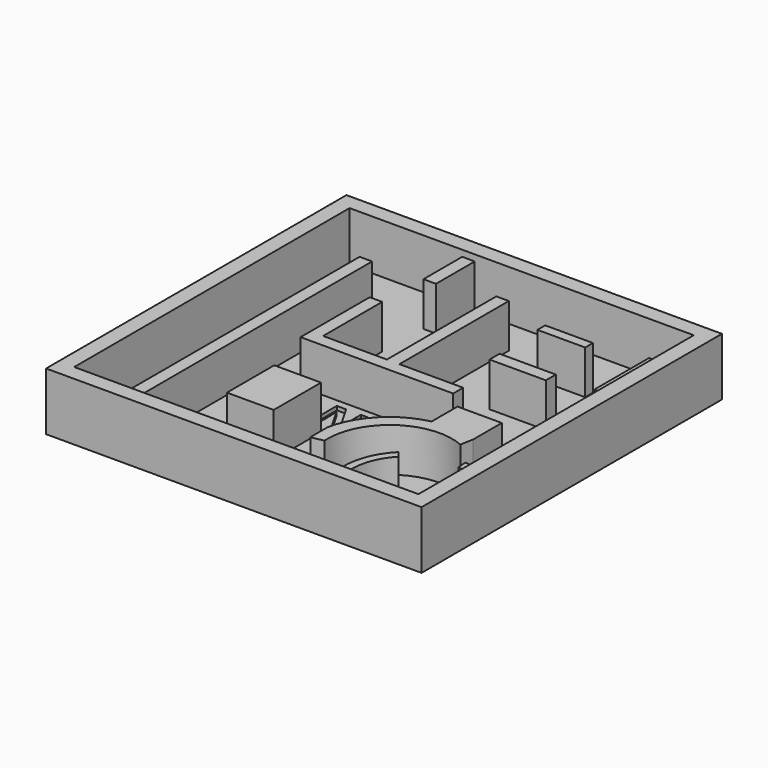
from build123d import *

# Parameters (mm, degrees)
F0_W         = 38.1
F0_H         = 38.1
F1_DEPTH     = 0.79375
F2_W         = 38.1
F2_H         = 38.1
F2_W_2       = 34.925
F2_H_2       = 34.925
F3_DEPTH     = 5.08
F5_TEXT_SIZE = 4.9165669932
F6_DEPTH     = 0.396875
F7_R         = 1.27
F8_DEPTH     = 0.396875
F9_R         = 1.27
F10_DEPTH    = 0.396875
F4_W         = 1.27
F4_H         = 29.845
F4_H_2       = 4.9190903239
F4_W_2       = 4.8410449686
F4_H_3       = 0.9841924552
F4_W_3       = 5.715
F4_H_4       = 1.27
F4_W_4       = 4.7475340998
F4_H_5       = 6.0008075448
F11_DEPTH    = 4.445
F12_W        = 1.0896102858
F12_H        = 6.9149732516
F13_DEPTH    = 4.445


# Not quite as in the source:
# - Text() gives the source's letters only with a copy of the font that has no kerning and outlines rounded to 1/6400 em; it was checked with that copy


with BuildPart() as f1:
    # F0 (on Top) → F1 (new body)
    with BuildSketch(Plane.XY):
        with Locations((1.1348947883, -10.0670298852)):
            Rectangle(F0_W, F0_H)
    extrude(amount=F1_DEPTH)

    # F2 (on face) → F3 (join)
    with BuildSketch(Plane.XY.offset(0.79375)):
        with Locations((1.1348947883, -10.0670298852)):
            Rectangle(F2_W, F2_H)
        with Locations((1.1348947883, -10.0670298852)):
            Rectangle(F2_W_2, F2_H_2, mode=Mode.SUBTRACT)
    extrude(amount=F3_DEPTH)

    # F5 (on face) → F6 (cut)
    with BuildSketch(Plane.XY.offset(0.79375)):
        with Locations((-2.4528526701, -15.6311374158)):
            Text('NB', F5_TEXT_SIZE, font='Open Sans', font_style=FontStyle.BOLD, text_align=(TextAlign.LEFT, TextAlign.BOTTOM))
    extrude(amount=-F6_DEPTH, mode=Mode.SUBTRACT)

    # F7 (on face) → F8 (cut)
    with BuildSketch(Plane.XY.offset(0.79375)):
        with Locations((-13.7639371678, -25.5260914564)):
            Circle(F7_R)
    extrude(amount=-F8_DEPTH, mode=Mode.SUBTRACT)

    # F9 (on face) → F10 (cut)
    with BuildSketch(Plane.XY.offset(0.79375)):
        with Locations((15.1944022471, -24.998095862)):
            Circle(F9_R)
    extrude(amount=-F10_DEPTH, mode=Mode.SUBTRACT)

    # F4 (on face) → F11 (join)
    with BuildSketch(Plane.XY.offset(0.79375)):
        with Locations((-10.6126052117, -12.6070298852)):
            Rectangle(F4_W, F4_H)
        Polygon((1.4523947883, -10.0987223404), (-5.0191486603, -10.0987223404), (-5.0191486603, -2.6036202091), (-6.2891486603, -2.6036202091), (-6.2891486603, -10.0987223404), (-6.2891486603, -11.3687223404), (-2.2360617632, -11.3687223404), (9.1939382368, -11.3687223404), (9.1939382368, -10.0987223404), (2.7223947883, -10.0987223404), (2.7223947883, 3.7798983976), (1.4523947883, 3.7798983976), align=None)
        with Locations((-4.2626052117, 4.9359249528)):
            Rectangle(F4_W, F4_H_2)
        with Locations((10.0072620182, 1.8233738872)):
            Rectangle(F4_W_2, F4_H_3)
        with Locations((10.6598947883, -4.3837223404)):
            Rectangle(F4_W_3, F4_H_4)
        with BuildLine():
            ThreePointArc((10.8646293997, -16.187399974), (13.1387566838, -16.0284903217), (15.3588872355, -16.5461074727))
            Line((15.3588872355, -16.5461074727), (15.3588872355, -15.1834999244))
            Line((15.3588872355, -15.1834999244), (15.3588872355, -12.9101296591))
            Line((15.3588872355, -12.9101296591), (10.8646293997, -12.9101296591))
            Line((10.8646293997, -12.9101296591), (10.8646293997, -16.187399974))
        make_face()
        with BuildLine():
            Line((15.1174844813, -17.8607980719), (15.3588872355, -16.5461074727))
            ThreePointArc((15.3588872355, -16.5461074727), (13.1387566838, -16.0284903217), (10.8646293997, -16.187399974))
            ThreePointArc((10.8646293997, -16.187399974), (7.0862136004, -18.275880811), (5.0380298088, -22.0762914882))
            Line((5.0380298088, -22.0762914882), (5.0380298088, -24.2933216408))
            Line((5.0380298088, -24.2933216408), (6.2862870532, -24.0593262309))
            ThreePointArc((6.2862870532, -24.0593262309), (8.9633574039, -18.4831374981), (15.1174844813, -17.8607980719))
        make_face()
        with Locations((-2.5238381618, -19.4491261128)):
            Rectangle(F4_W_4, F4_H_5)
        with BuildLine():
            ThreePointArc((12.0882324968, -21.9232072916), (10.5199007092, -24.51182924), (10.2872829897, -27.5295298852))
            Line((10.2872829897, -27.5295298852), (11.0548400558, -27.5295298852))
            Line((11.0548400558, -27.5295298852), (11.0104987289, -26.9383224419))
            ThreePointArc((11.0104987289, -26.9383224419), (11.3299295677, -24.5747940823), (12.5820940698, -22.544920582))
            Line((12.5820940698, -22.544920582), (12.0882324968, -21.9232072916))
        make_face()
        with BuildLine():
            ThreePointArc((17.4170570996, -20.9862248128), (18.0148385759, -21.0932678026), (18.5973947883, -21.2648170798))
            Line((18.5973947883, -21.2648170798), (18.5973947883, -21.2593718124))
            Line((18.5973947883, -21.2593718124), (18.5973947883, -20.2500168551))
            ThreePointArc((18.5973947883, -20.2500168551), (17.9883820139, -20.1003730355), (17.3678223351, -20.0098439404))
            Line((17.3678223351, -20.0098439404), (17.4170570996, -20.9862248128))
        make_face()
    extrude(amount=F11_DEPTH)

    # F12 (on face) → F13 (join)
    with BuildSketch(Plane.XY.offset(0.79375)):
        with Locations((18.0525896454, -0.3800038211)):
            Rectangle(F12_W, F12_H)
    extrude(amount=F13_DEPTH)


solid = f1.part
